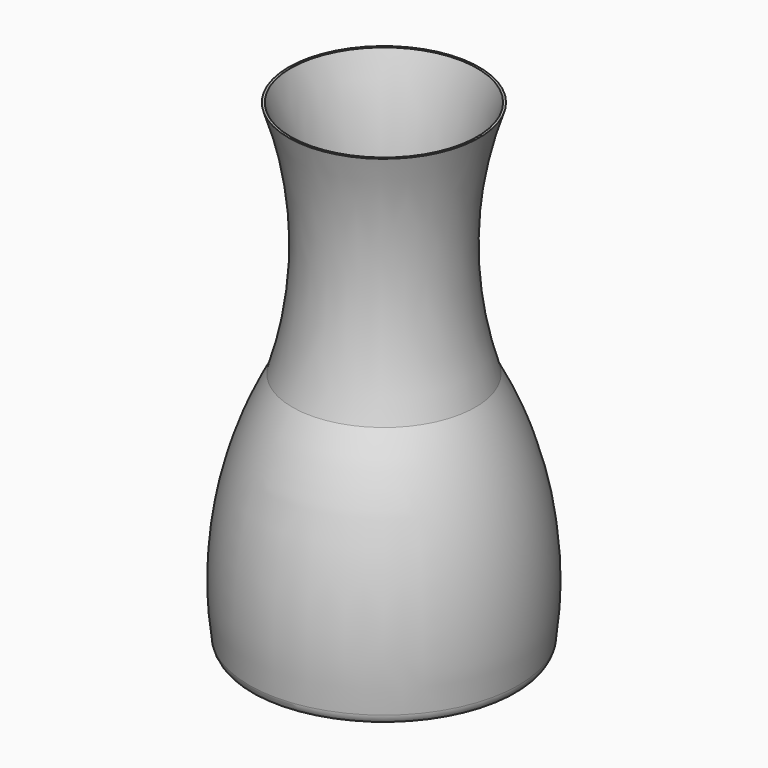
from build123d import *


# Not quite as in the source:
# - a fillet or chamfer that OpenCascade refuses, or shapes differently, is made with other operations: its cross-section is extruded or revolved along the edge and cut away or added


with BuildPart() as f1:
    # F0 (on Front) → F1 (revolve)
    with BuildSketch(Plane.XZ):
        with BuildLine():
            Line((-30.48, 79.375), (-29.718, 79.375))
            ThreePointArc((-29.718, 79.375), (-23.8719193553, 119.1661972903), (-30.988, 158.75))
            Line((-30.988, 158.75), (-31.75, 158.75))
            ThreePointArc((-31.75, 158.75), (-24.6339195933, 119.1661972865), (-30.48, 79.375))
        make_face()
        with BuildLine():
            Line((-44.45, 0), (-43.688, 0))
            ThreePointArc((-43.688, 0), (-43.2448466189, 40.8388650049), (-29.718, 79.375))
            Line((-29.718, 79.375), (-30.48, 79.375))
            ThreePointArc((-30.48, 79.375), (-44.0068462925, 40.8388649475), (-44.45, 0))
        make_face()
    revolve(axis=Axis((0, 0, 79.375), (0, 0, 1)))

    # F2: fillet of radius 5.08 on 1 edges, made by hand

    # F2_s1 → F2_t2 (revolve, cut)
    with BuildSketch(Plane.XZ):
        with BuildLine():
            ThreePointArc((-44.8195429295, 2.5826020544), (-44.4365427465, 1.2112215), (-43.688, 0))
            Line((-43.688, 0), (-44.45, 0))
            ThreePointArc((-44.45, 0), (-44.6414794787, 1.2903411816), (-44.8195429295, 2.5826020544))
        make_face()
    revolve(axis=Axis((0, 0, 0), (0, 0, 1)), mode=Mode.SUBTRACT)


solid = f1.part
